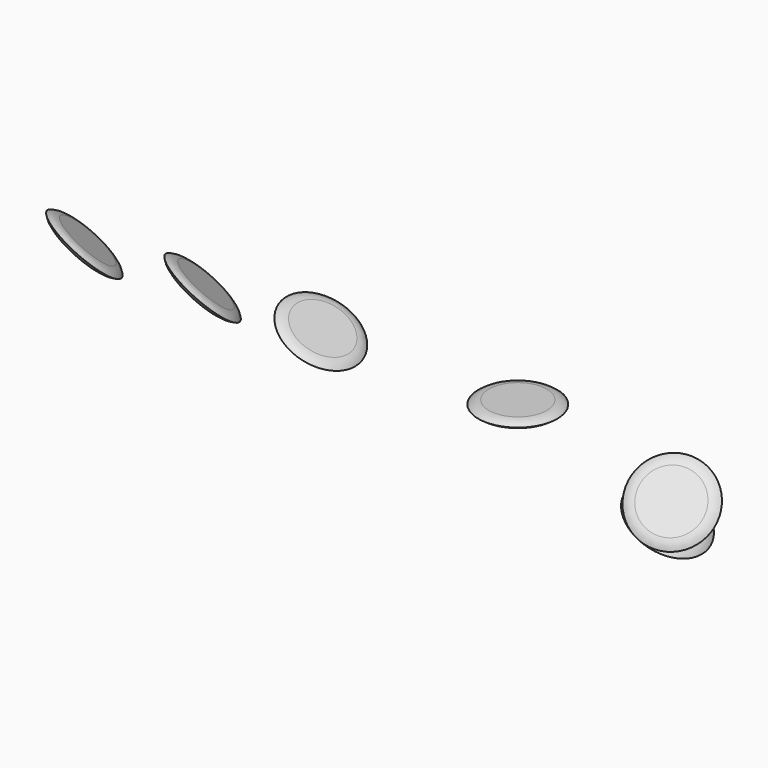
from build123d import *

# Parameters (mm, degrees)
F0_R      = 12.7
F1_DEPTH  = 1.27
F2_SIZE   = 1.26999
F8_ANGLE  = -30
F11_ANGLE = -45
F15_ANGLE = 30
F19_ANGLE = -30


# Not quite as in the source:
# - a fillet or chamfer that OpenCascade refuses, or shapes differently, is made with other operations: its cross-section is extruded or revolved along the edge and cut away or added
# - a fillet or chamfer is up to 0.001 mm smaller than in the source, because OpenCascade refuses the exact size


with BuildPart() as f1:
    # F0 (on Top) → F1 (new body, symmetric)
    with BuildSketch(Plane.XY):
        Circle(F0_R)
    extrude(amount=F1_DEPTH, both=True)

    # F2 (size 1.27 in the source; OpenCascade refuses exactly that, so slightly less here)
    f2_edges = [f1.edges().sort_by_distance(p)[0] for p in [
        (-12.7, 0, -1.27),
        (-12.7, 0, 1.27),
    ]]
    chamfer(f2_edges, length=F2_SIZE)

    # F3: fillet of radius 5.08 on 1 edges, made by hand

    # F3_s1 → F3_t2 (revolve, cut)
    with BuildSketch(Plane.XZ):
        with BuildLine():
            ThreePointArc((12.7, 1e-05), (11.135951327, 0.9419075538), (9.3399071739, 1.27))
            Line((9.3399071739, 1.27), (11.43001, 1.27))
            Line((11.43001, 1.27), (12.7, 1e-05))
        make_face()
    revolve(axis=Axis((0, 0, 1.27), (0, 0, 1)), mode=Mode.SUBTRACT)

    # F4: fillet of radius 5.08 on 1 edges, made by hand

    # F4_s1 → F4_t2 (revolve, cut)
    with BuildSketch(Plane.XZ):
        with BuildLine():
            ThreePointArc((12.7, -1e-05), (11.135951327, -0.9419075538), (9.3399071739, -1.27))
            Line((9.3399071739, -1.27), (11.43001, -1.27))
            Line((11.43001, -1.27), (12.7, -1e-05))
        make_face()
    revolve(axis=Axis((0, 0, -1.27), (0, 0, 1)), mode=Mode.SUBTRACT)


with BuildPart() as f5_1:
    # F5: copy of F1
    add(f1.part.moved(Location((38.1, 12.7, -25.4))))


with BuildPart() as f5_1_1:
    # F8: moved
    add(f5_1.part.rotate(Axis((38.1, 17.4700720236, -25.4), (0, -1, 0)), F8_ANGLE))


with BuildPart() as f11_1:
    # F11: copy of F5_1
    add(f5_1_1.part.rotate(Axis((33.3806926878, 0, -22.6753066529), (-0.8660254038, 0, 0.5)), F11_ANGLE))


with BuildPart() as f12_1:
    # F12: copy of F1
    add(f1.part.moved(Location((-63.5, 0, 0))))


with BuildPart() as f12_1_1:
    # F15: moved
    add(f12_1.part.rotate(Axis((-63.5, 5.5880947039, 0), (0, 1, 0)), F15_ANGLE))


with BuildPart() as f16_1:
    # F16: copy of F12_1
    add(f12_1_1.part.moved(Location((-38.1, 0, 0))))


with BuildPart() as f16_1_1:
    # F19: moved
    add(f16_1.part.rotate(Axis((-103.8624103101, 0, 1.3062032016), (0.8660254038, 0, -0.5)), F19_ANGLE))


with BuildPart() as f20_1:
    # F20: copy of F16_1
    add(f16_1_1.part.moved(Location((-38.1, 0, 0))))


solid = Compound([f1.part, f5_1_1.part, f11_1.part, f12_1_1.part, f16_1_1.part, f20_1.part])
